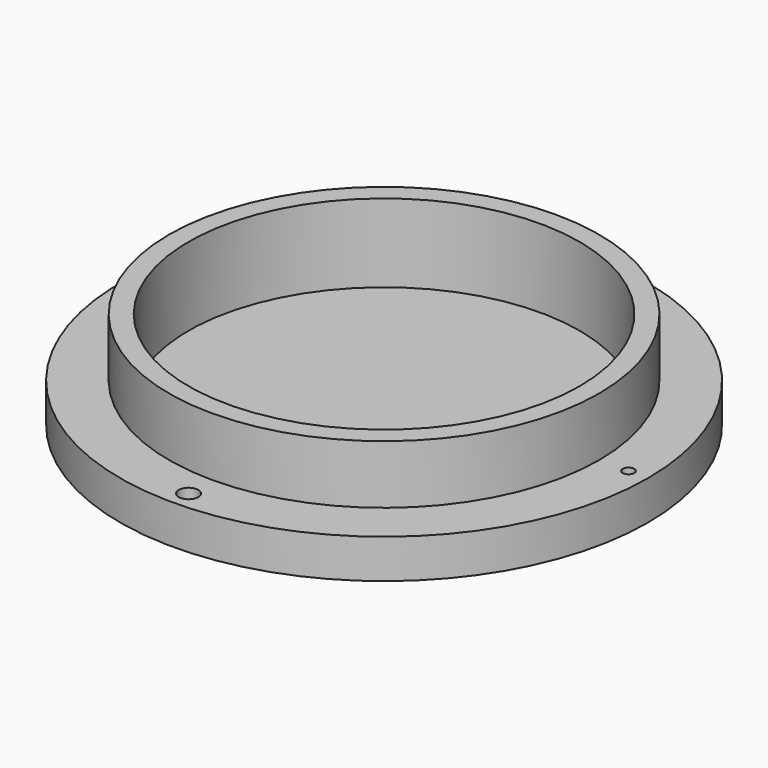
from build123d import *

# Parameters (mm, degrees)
F0_R     = 11
F1_DEPTH = 5
F0_R_2   = 13.5
F2_DEPTH = 2
F3_T     = 1
F4_R     = 0.3407547834
F4_R_2   = 0.295229786
F4_R_3   = 0.330794191
F4_R_4   = 0.5
F5_DEPTH = 126.8


# Not quite as in the source:
# - a shell that OpenCascade refuses in one call is made with other operations: the cavity is built on its own and cut out


with BuildPart() as f1:
    # F0 (on Top) → F1 (new body)
    with BuildSketch(Plane.XY):
        Circle(F0_R)
    extrude(amount=F1_DEPTH)

    # F0 (on Top) → F2 (join)
    with BuildSketch(Plane.XY):
        Circle(F0_R_2)
        Circle(F0_R, mode=Mode.SUBTRACT)
    extrude(amount=F2_DEPTH)

    # F3: shell of thickness 1, made by hand


with BuildPart() as f3_core1:
    # F3_t2: copy of F1
    add(f1.part)

    # the walls: a layer under each face that stays
    f3_faces = [f3_core1.faces().sort_by_distance(p)[0] for p in [
        (-11, 0, 3.5),
        (-9, -9, 2),
        (-13.5, 0, 1),
        (0, 0, 0),
    ]]
    thicken(f3_faces, amount=-F3_T, mode=Mode.SUBTRACT)

    # F3_s3 → F3_t4 (revolve, cut)
    with BuildSketch(Plane.XZ):
        Polygon((11.01, 2.01), (10, 2), (10, 1), (11, 1), align=None)
    revolve(axis=Axis((0, 0, 2), (0, 0, 1)), mode=Mode.SUBTRACT)


with BuildPart() as f1_1:
    add(f1.part)

    # what is left inside the walls is the cavity
    f3_cavity = [f3_core1.part.solids().sort_by_distance(p)[0] for p in [
        (0, -3.333333, 1.01),
    ]]
    add(f3_cavity, mode=Mode.SUBTRACT)

    # F4 (on face) → F5 (cut, symmetric)
    with BuildSketch(Plane.XY):
        with Locations((-12.5, 0)):
            Circle(F4_R)
        with Locations((12.5, 0)):
            Circle(F4_R_2)
        with Locations((0, 12.5)):
            Circle(F4_R_3)
        with Locations((0, -12.5)):
            Circle(F4_R_4)
    extrude(amount=F5_DEPTH, both=True, mode=Mode.SUBTRACT)


solid = f1_1.part
